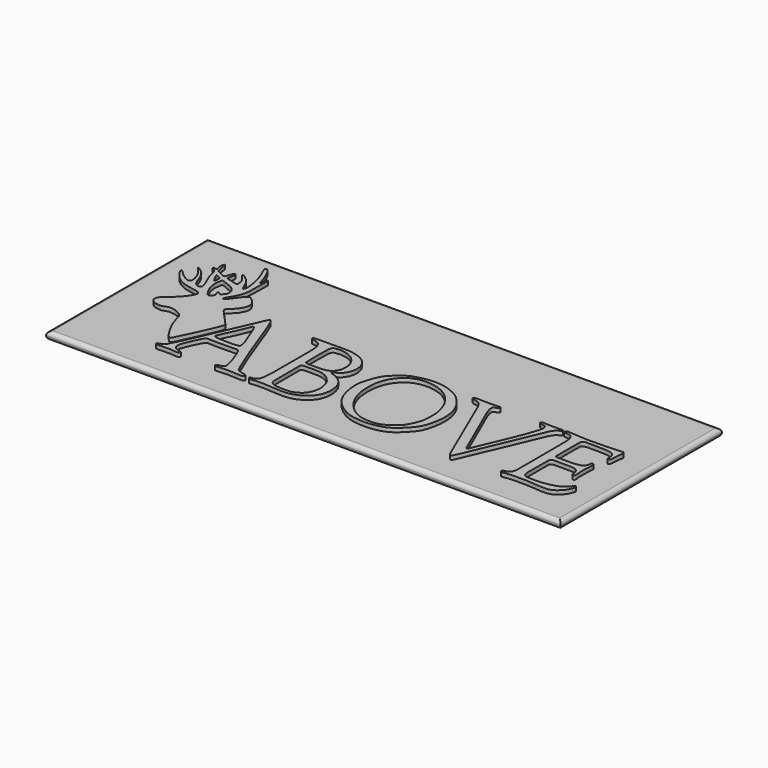
from build123d import *

# Parameters (mm, degrees)
F1_DEPTH = 0.4
F3_DEPTH = 2
F4_W     = 130.9761814773
F4_H     = 51.3558490202
F5_DEPTH = 1
F6_R     = 0.99999
F7_DEPTH = 2


# Not quite as in the source:
# - a fillet or chamfer is up to 0.001 mm smaller than in the source, because OpenCascade refuses the exact size


with BuildPart() as f1:
    # F0 (on Top) → F1 (new body)
    with BuildSketch(Plane.XY):
        with BuildLine():
            add(Edge.make_bspline(
                [(-15.2332797082, -10.2984596184), (-15.0093942884, -9.6524336301), (-15.0840574343, -9.1280532888), (-19.4655234335, -4.9444968794), (-19.1923468425, -4.0814513582), (-17.0227818195, -2.3777963682), (-15.9772713992, 0.6445409531), (-17.9010980306, 2.3727251331), (-19.2227726204, 3.4732306517), (-22.0102515264, -1.694371511), (-22.675957849, -0.7190837107), (-21.4698886603, 0.7632452243), (-20.1707249074, 3.6211502447), (-20.3340098043, 7.3677276696), (-20.0693177036, 11.1555273847), (-20.7490299306, 10.0046641789), (-20.7993278871, 7.9484959257), (-21.6196261476, 11.7801006923), (-23.3189903301, 14.5604952951), (-24.2268096177, 14.163796693), (-22.3143449492, 11.0669257332), (-21.331542924, 5.6400698523), (-22.149053501, 4.2936073138), (-22.8841040318, 7.5286045669), (-25.190165698, 9.3200917664), (-26.0899436297, 9.4842529604), (-24.1985357481, 7.5014652247), (-24.0857988599, 6.3361531301), (-24.1034586627, 5.3123553051), (-26.1386607352, 6.1357702948), (-27.122761487, 6.2654212324), (-27.2973682829, 6.6475846064), (-26.710529351, 8.7559265568), (-27.5771616457, 8.8747247494), (-27.9381930899, 6.9693446297), (-28.3530093382, 6.4188046355), (-30.1959305266, 7.4880147192), (-30.6145836041, 7.6246936128), (-31.1504494343, 9.4485056194), (-31.0918334587, 11.0700867085), (-31.8428582792, 9.7455582197), (-31.0093663734, 7.608908434), (-31.9606356015, 8.4144559492), (-32.5662439462, 7.9809408066), (-30.8829651102, 7.3675040083), (-31.1062693781, 5.1768624873), (-27.8910672871, -0.2497095271), (-31.266558052, 0.2817087175), (-31.6391364369, 4.8260598868), (-35.8656403415, 7.148054973), (-32.5956541042, 4.5606439482), (-31.5129435253, -0.6532739833), (-35.3555837278, 2.3321158484), (-35.5396776514, 2.6488410814), (-37.423089105, 4.3576754946), (-34.149133245, -1.644392368), (-27.3820098453, -1.2956673683), (-27.8794549907, -3.5887880219), (-30.3693556852, -6.6236284339), (-33.142877036, -8.3616003025), (-33.1843468192, -10.5862835101), (-29.9525050745, -11.479426381), (-28.7488139728, -10.1627989737), (-24.3130688974, -11.3403488056), (-24.3577602886, -14.9079605545), (-20.408517341, -21.5471299333), (-19.3708138898, -19.6570120394), (-15.8667838924, -12.1264489854), (-15.2332797082, -10.2984596184)],
                knots=[0, 0, 0, 0, 0.0120407609, 0.0369548453, 0.0455998656, 0.0626817696, 0.0806453343, 0.096699598, 0.1079623462, 0.131302389, 0.1377707175, 0.1515788078, 0.1702063006, 0.1919656057, 0.2094349262, 0.2180452799, 0.2292360252, 0.2468462896, 0.2660436632, 0.2722493285, 0.291374186, 0.316870226, 0.3253231285, 0.3424600791, 0.3610099087, 0.3669824396, 0.382641769, 0.394942166, 0.4030509241, 0.417573897, 0.4280639686, 0.4342264289, 0.4491088709, 0.4554393353, 0.4696299423, 0.4773554298, 0.4919040126, 0.4992434437, 0.5138107783, 0.5247485618, 0.5349387212, 0.5487104407, 0.5571075282, 0.5634453361, 0.5747861505, 0.5909866388, 0.6145658117, 0.6271821922, 0.6498661243, 0.6673736433, 0.6844679828, 0.7042723063, 0.7225110601, 0.7315999829, 0.7424569843, 0.7648776789, 0.7908505506, 0.8029463447, 0.824154807, 0.8430628881, 0.856291921, 0.8737242258, 0.8873169312, 0.907208903, 0.9275153958, 0.9544482361, 0.9659295704, 1, 1, 1, 1], degree=3))
        make_face()
        with BuildLine():
            add(Edge.make_bspline(
                [(-29.7977950352, 6.2162249849), (-29.7993964975, 6.0210812953), (-28.825569652, 3.8423834775), (-28.4519385095, 4.1422737352), (-28.3900703312, 5.1631622895), (-28.373725171, 5.5205005946), (-29.5818671337, 6.0474269447), (-29.7973504539, 6.2703987425), (-29.7977950352, 6.2162249849)],
                knots=[0, 0, 0, 0, 0.299300632, 0.3869764424, 0.5805649542, 0.6945409912, 0.9169112775, 1, 1, 1, 1], degree=3))
        make_face(mode=Mode.SUBTRACT)
        with BuildLine():
            add(Edge.make_bspline(
                [(-27.4534161738, 4.8815971646), (-27.5829006668, 4.6197704851), (-27.8833951504, 2.8656868488), (-27.3925534695, 0.799538413), (-26.4658323416, -0.8375371732), (-25.8457754123, -1.7123795224), (-25.2731466356, -1.7150173269), (-24.6325995931, -0.8642885968), (-24.6173490595, -0.6062435916), (-24.9744846122, 0.1084179836), (-24.9952901889, 0.8322824569), (-24.1482202231, 0.0273024167), (-23.7244798154, 0.3033967102), (-22.9372055408, 1.1829986707), (-23.0915123982, 2.4562011894), (-23.8408625303, 3.8662768208), (-26.9223285545, 4.8960420358), (-27.3223330185, 5.0270299743), (-27.4145706618, 4.9601455004), (-27.4534161738, 4.8815971646)],
                knots=[0, 0, 0, 0, 0.0817632462, 0.1726013597, 0.2550012881, 0.3138554901, 0.3543569034, 0.4137592441, 0.444060647, 0.4986368209, 0.5368103458, 0.5910850521, 0.630502456, 0.6931495414, 0.7578834718, 0.8336767969, 0.9399672197, 0.9754709225, 1, 1, 1, 1], degree=3))
        make_face(mode=Mode.SUBTRACT)
    extrude(amount=F1_DEPTH)


with BuildPart() as f3:
    # F2 (on Top) → F3 (new body)
    with BuildSketch(Plane.XY):
        with BuildLine():
            add(Edge.make_bspline(
                [(-17.8186707199, -24.5789550245), (-18.5262242711, -24.6304439452), (-20.358175603, -24.7394529453), (-20.7940909596, -24.4840161854), (-20.6337741479, -23.9779671505), (-19.3896907217, -23.8896324628), (-18.1771791891, -22.2724269857), (-9.970002365, -3.1502325051), (-9.4341293462, -2.1626326794), (-8.5298213567, -3.0073907103), (-6.1164796385, -10.2539467622), (-1.3806819347, -22.3025182489), (-0.683738408, -23.2547899839), (0.586258441, -23.6686196362), (1.6564266278, -23.8527715304), (1.9065968781, -24.3190250875), (1.4282647943, -24.8392161885), (-2.5654340217, -24.2992923004), (-5.0926669543, -24.6635461429), (-5.6461058536, -24.609920481), (-5.8601113726, -24.1039841591), (-4.9881206956, -23.8322315995), (-4.0057600347, -23.7565204031), (-3.7041440652, -22.3979584639), (-5.970768949, -16.3593958047), (-6.6672962176, -16.3671332574), (-13.9351018709, -16.5336977205), (-14.4412111372, -16.1030933493), (-17.1251492443, -21.5812553775), (-16.8820571682, -23.0099438036), (-16.3728003844, -23.6025789105), (-15.1423881637, -24.1280540106), (-14.5677091572, -24.0823658212), (-14.4953555678, -24.9679629884), (-16.8880971826, -24.4933044304), (-17.3513145138, -24.544945349), (-17.8186707199, -24.5789550245)],
                knots=[0, 0, 0, 0, 0.034606547, 0.0478551254, 0.0607316403, 0.0815592174, 0.1138190862, 0.2124412902, 0.2309948002, 0.2485416257, 0.3094963798, 0.3875252451, 0.409110504, 0.433162012, 0.4555813572, 0.4688299488, 0.4829975336, 0.5262737256, 0.5615253264, 0.5756929131, 0.588282433, 0.6072660436, 0.6274333282, 0.6509110315, 0.7042405462, 0.7242470082, 0.7812023235, 0.7974767625, 0.8486624145, 0.8746413843, 0.8926317285, 0.9174233866, 0.9324998026, 0.9465406554, 0.9771415401, 1, 1, 1, 1], degree=3))
        make_face()
        with BuildLine():
            add(Edge.make_bspline(
                [(-10.6451269239, -7.6531427912), (-11.1635320486, -9.140155094), (-13.5771506003, -13.9866832023), (-13.6553005281, -14.612677821), (-13.1015114277, -15.08954204), (-6.8594531157, -15.1835333702), (-7.1281559565, -14.448692861), (-7.09391842, -13.2187966821), (-8.656445023, -9.9815808182), (-9.7266075902, -6.5997926543), (-10.4475039943, -6.7365001924), (-10.4546387692, -7.1067395708), (-10.6451269239, -7.6531427912)],
                knots=[0, 0, 0, 0, 0.1955711938, 0.2489704346, 0.3074664099, 0.4860203681, 0.5291103449, 0.6060239634, 0.7520174877, 0.8858844196, 0.9281372925, 1, 1, 1, 1], degree=3))
        make_face(mode=Mode.SUBTRACT)
    extrude(amount=F3_DEPTH)


with BuildPart() as f3b:
    # F2 (on Top) → F3, piece 2 (new body)
    with BuildSketch(Plane.XY):
        with BuildLine():
            add(Edge.make_bspline(
                [(2.9986717273, -2.9176652897), (4.5731932325, -2.8947406218), (10.9523054272, -2.8056420795), (11.8491369393, -2.9704794263), (15.1441637743, -3.7111802915), (17.1291392253, -5.973921605), (17.4434691373, -8.7077246139), (16.351884791, -11.3349808797), (14.4830876864, -12.0868741598), (14.2065407888, -12.6919101169), (15.3907005999, -12.7503578443), (18.0051408366, -14.3724783841), (18.9323318972, -16.612656188), (19.2045201156, -19.8438815811), (17.5618176451, -22.9328146445), (14.4991929645, -24.5620027924), (11.9328529247, -24.9275981507), (8.0759131802, -24.6237266642), (5.2376508672, -24.4574170198), (3.4847200578, -24.7552756049), (3.000104703, -24.6856083566), (2.840094494, -24.2661535545), (3.1077172317, -23.9845093652), (3.7233931441, -24.1261225507), (4.8130212078, -23.4964830947), (5.1143694454, -21.7499883345), (5.2795577601, -18.7920313061), (5.093980589, -12.2053829442), (5.3207697442, -7.2503768517), (4.9675852293, -5.2741108501), (4.518908773, -4.3142462301), (3.4077663416, -3.6151473735), (2.4609358883, -3.7162434327), (2.047195786, -3.4704848142), (2.1544159455, -2.9304379219), (2.4815498265, -2.9251944646), (2.9986717273, -2.9176652897)],
                knots=[0, 0, 0, 0, 0.0594003701, 0.0835026048, 0.1206841975, 0.1572307632, 0.1917765774, 0.2270665321, 0.256394898, 0.2691563441, 0.2892990909, 0.3263944414, 0.3595571245, 0.3971334828, 0.4362595917, 0.4749411121, 0.5094013726, 0.5512949807, 0.5882689746, 0.6158124967, 0.6294268394, 0.6421580801, 0.6537191257, 0.6698855437, 0.6922755626, 0.7193150847, 0.7560647655, 0.811759297, 0.8599220026, 0.8888715544, 0.9100993257, 0.9338553359, 0.9544697139, 0.9676822069, 0.9804910684, 1, 1, 1, 1], degree=3))
        make_face()
        with BuildLine():
            add(Edge.make_bspline(
                [(7.9134525731, -13.5765336454), (8.4656908215, -13.5249837722), (12.0166451852, -13.482074654), (13.1072424292, -13.7143378792), (14.509090113, -14.3336197357), (15.6591165801, -15.5440421064), (16.1790934207, -16.2740694615), (16.7715367956, -18.0506637137), (16.81110186, -19.5984971483), (16.3535796726, -21.4566097884), (15.4796202328, -22.7291384826), (13.9450284962, -23.653515414), (12.4734478276, -24.0015308029), (9.9325274889, -23.9052985449), (8.9655494456, -23.7359270018), (8.2751637862, -23.4966310779), (7.5920920663, -22.8790822924), (7.5227255198, -21.8494720153), (7.5755301319, -17.2633260081), (7.5553347596, -14.0348315189), (7.5658004299, -13.885882511), (7.708510426, -13.617057364), (7.7812264073, -13.5888765827), (7.9134525731, -13.5765336454)],
                knots=[0, 0, 0, 0, 0.0796721885, 0.1263040133, 0.1742904671, 0.225547667, 0.2640510909, 0.3176224, 0.3685996925, 0.4231997985, 0.472914118, 0.5250153616, 0.5755784316, 0.6391972187, 0.6790868472, 0.7126185496, 0.7487122899, 0.7874658877, 0.8765007975, 0.9467593746, 0.960892758, 0.9809235452, 1, 1, 1, 1], degree=3))
        make_face(mode=Mode.SUBTRACT)
        with BuildLine():
            add(Edge.make_bspline(
                [(7.5597460382, -5.1983157173), (7.5768174771, -4.7752658686), (7.6117939175, -4.5599184391), (7.8915823244, -3.9518990986), (8.5512243646, -3.7987113384), (9.6421145995, -3.6374130657), (12.0142479626, -4.0121152092), (13.9056770375, -5.3663836659), (15.0189228434, -7.2511220165), (15.1903015952, -9.0285684555), (14.9912671632, -10.3350820672), (14.3210946635, -11.493000004), (13.0422817282, -12.5872460163), (8.3767248185, -12.4282745943), (7.9626085673, -12.42584987), (7.6082300578, -12.2055804985), (7.4622628161, -11.7055791022), (7.5083058526, -6.4730625476), (7.5597460382, -5.1983157173)],
                knots=[0, 0, 0, 0, 0.04366644, 0.0812507687, 0.1215889048, 0.1754155404, 0.2545074138, 0.3331504508, 0.4083572449, 0.4764587283, 0.5350867206, 0.5920341657, 0.6594086428, 0.7688242446, 0.8023163354, 0.8306341757, 0.8684229384, 1, 1, 1, 1], degree=3))
        make_face(mode=Mode.SUBTRACT)
    extrude(amount=F3_DEPTH)


with BuildPart() as f3c:
    # F2 (on Top) → F3, piece 3 (new body)
    with BuildSketch(Plane.XY):
        with BuildLine():
            add(Edge.make_bspline(
                [(31.6981896758, -2.7517566923), (32.4855511917, -2.6662951361), (33.6973140893, -2.686447277), (35.4124903207, -2.8976716178), (37.365271922, -3.487745744), (39.7322577308, -4.6286347181), (41.7448723321, -6.7403695787), (42.9307226187, -8.5981241795), (43.7743743926, -11.0623168107), (44.0310311172, -14.1276205282), (43.2370107981, -18.0437680394), (42.1417511843, -20.2200499423), (39.0584845813, -23.3581879437), (36.6879540703, -24.4147562849), (33.547977925, -25.0431152226), (29.8149106979, -24.7845936888), (27.2978257333, -24.0149400802), (24.1855473843, -21.8152677053), (22.3600004098, -19.1779329614), (21.4690708366, -15.8722935856), (21.327289014, -13.3523817345), (21.5138448111, -11.6902719815), (22.6387088646, -8.2258594008), (23.7475713067, -6.6545022043), (26.1812598582, -4.3383661288), (28.3603805442, -3.356356178), (30.6942257638, -2.8607286405), (31.6981896758, -2.7517566923)],
                knots=[0, 0, 0, 0, 0.0341965483, 0.0650580209, 0.0990248333, 0.1379292236, 0.1785675923, 0.2140382543, 0.2519077228, 0.2943765314, 0.34143948, 0.3795504523, 0.428692638, 0.4674522524, 0.5099281851, 0.5559166818, 0.5949378648, 0.6407882758, 0.6838578711, 0.7280535962, 0.765304292, 0.7967660624, 0.8414591274, 0.8758812293, 0.9184921551, 0.9563960141, 1, 1, 1, 1], degree=3))
        make_face()
        with BuildLine():
            add(Edge.make_bspline(
                [(32.3757380247, -3.7556143943), (33.2958323259, -3.835045558), (35.3374829386, -4.2298619022), (37.8702307643, -5.7717201967), (39.5353026217, -7.7515539991), (40.6118543591, -9.4957685202), (41.3311781149, -11.9217308369), (41.537384592, -13.2175494886), (41.5631804343, -16.024805783), (41.3191550954, -17.6196524909), (40.0632173963, -20.4459911485), (39.0176525098, -21.7261039941), (36.4226916998, -23.6310371312), (34.2590014297, -24.0790860379), (31.240481395, -23.9596385587), (29.4134002337, -23.1742800285), (27.5909988603, -22.0154832916), (25.8072628968, -19.8685430648), (24.9790822222, -18.3822532534), (24.1095178811, -16.0311551863), (23.9312299748, -14.4145168967), (23.7957549823, -12.4832029945), (23.9334985957, -10.5232236657), (24.6149450631, -8.233839022), (25.2694976229, -7.0783307387), (26.3486933371, -5.6845001426), (27.7015348542, -4.5304110567), (30.0674452085, -3.7306413055), (31.5570074754, -3.6849338998), (32.3757380247, -3.7556143943)],
                knots=[0, 0, 0, 0, 0.0429022088, 0.0858322177, 0.1254390468, 0.1616438754, 0.200344307, 0.2299741373, 0.2705942497, 0.3038292435, 0.3463741966, 0.3795926892, 0.4230236918, 0.4608566752, 0.5034618232, 0.5384774913, 0.5750783278, 0.6162288942, 0.6495270762, 0.6883054272, 0.720542142, 0.7546314557, 0.7902429882, 0.8283403313, 0.8573019616, 0.8897134595, 0.9230753544, 0.9618241859, 1, 1, 1, 1], degree=3))
        make_face(mode=Mode.SUBTRACT)
    extrude(amount=F3_DEPTH)


with BuildPart() as f3d:
    # F2 (on Top) → F3, piece 4 (new body)
    with BuildSketch(Plane.XY):
        with BuildLine():
            add(Edge.make_bspline(
                [(43.4478521587, -3.0493328889), (44.5846660798, -3.1063553315), (46.6244936083, -3.2085442718), (49.4442464963, -3.0121823146), (49.8430234234, -3.0347621192), (50.0485700829, -3.3512100722), (49.7660583429, -3.674682885), (49.3274870978, -3.7871947915), (48.8139123394, -4.0140117338), (48.5980931136, -4.4175614975), (48.7332427344, -5.3460822505), (49.3050834915, -6.9306989902), (51.1307713098, -10.9088610465), (55.2860542634, -20.5594377099), (55.3790988692, -20.7607972863), (55.3798365892, -20.760195779), (55.4215515437, -20.8339544375)],
                knots=[0, 0, 0, 0, 0.1188220262, 0.2237195129, 0.2608396256, 0.2948710905, 0.3332159131, 0.3773807578, 0.424501898, 0.4653824938, 0.5249451089, 0.6028688594, 0.749352672, 0.9539072272, 0.97311764, 0.9946758844, 0.9946758844, 0.9946758844, 0.9946758844], degree=3))
            add(Edge.make_bspline(
                [(55.4607037074, -20.9034150784), (55.4866189211, -20.9430088187), (55.5388381616, -21.022790335), (55.6560705125, -21.1784298749), (55.9305236933, -20.9984367057), (56.1392833118, -20.5234944666), (56.3837353272, -20.0621710379), (58.4718341466, -14.9666961091), (60.3944590747, -10.6123481531), (61.7502440603, -6.8328535787), (62.0979632028, -5.5929443597), (62.1938028184, -4.7472395828), (62.1227279981, -4.2320286696), (61.8320675007, -3.8800678569), (61.3656773155, -3.7644159671), (60.5629669431, -3.6089124364), (60.3459094201, -3.4920842872), (60.1055323717, -3.3316895125), (60.1372555353, -3.1150390963), (60.3239178294, -2.9576815651), (60.7711186994, -2.9102152421), (62.4420232453, -3.1033594688), (65.5839100323, -3.002560101), (65.6363353042, -2.9806084462), (65.9109486239, -3.081184096), (65.8590357012, -3.5015165095), (65.3542516668, -3.587012591), (64.4140603578, -4.2094095114), (63.7112014267, -5.5838872142), (62.804680902, -7.8958159046), (60.2703107713, -13.7714791057), (58.891988443, -17.0987199578), (57.4604076229, -20.3876905791), (55.9606004977, -23.932193809), (55.6045347914, -24.8074523644), (55.3690455445, -25.2644164156), (55.0818956105, -25.4798132289), (54.7062400575, -25.3298895913), (54.358648808, -24.742624418), (53.1783713435, -21.884382719), (52.1770231081, -19.5366299305), (51.0835176671, -17.0092270696), (49.7964172999, -14.04326035), (48.3314159163, -10.6108341908), (46.9299138991, -7.3547336689), (45.9859771758, -5.1659938333), (45.4431505429, -4.4583801964), (44.8930013483, -4.0178146836), (44.3657666742, -3.8838703949), (43.721768661, -3.7882978412), (43.2686629705, -3.6332026634), (43.1462142801, -3.5755733492), (43.0385249855, -3.2680682596), (43.2752626563, -3.0655793599), (43.3950395425, -3.0543043306), (43.4478521587, -3.0493328889)],
                knots=[0, 0, 0, 0, 0.0069195808, 0.0139429779, 0.0232181225, 0.0357670809, 0.048423783, 0.0893876317, 0.1316102802, 0.1668085072, 0.1869548417, 0.2030729985, 0.2158274826, 0.2272557348, 0.2399557033, 0.2561310963, 0.2653567827, 0.2743797104, 0.2820397862, 0.2903830247, 0.3012570035, 0.3261470545, 0.3574257754, 0.3617631056, 0.3703785591, 0.3804125429, 0.3925272533, 0.4112135027, 0.4329087196, 0.461589806, 0.5071989225, 0.5420687864, 0.5766617428, 0.6117707112, 0.6288917885, 0.6412497336, 0.6513234957, 0.6615107064, 0.6757756137, 0.7071612792, 0.7369589923, 0.7664511377, 0.7988955327, 0.8340077468, 0.8685372617, 0.8958968437, 0.9125277557, 0.9271130859, 0.9403499786, 0.9551753729, 0.9673602344, 0.9737678566, 0.983189181, 0.9925876907, 1, 1, 1, 1], degree=3))
            add(Edge.make_bspline(
                [(55.4215515437, -20.8339544375), (55.4318536462, -20.8521701892), (55.4446762067, -20.8749039801), (55.4607037074, -20.9034150784)],
                knots=[0.9946758844, 0.9946758844, 0.9946758844, 0.9946758844, 1, 1, 1, 1], degree=3))
        make_face()
    extrude(amount=F3_DEPTH)


with BuildPart() as f3e:
    # F2 (on Top) → F3, piece 5 (new body)
    with BuildSketch(Plane.XY):
        with BuildLine():
            add(Edge.make_bspline(
                [(67.0425593853, -2.8810673393), (67.8678731279, -2.938649076), (72.7499173271, -3.4609926409), (80.755809882, -2.9446053024), (80.9969352571, -2.8768406134), (81.5035604288, -3.2620983162), (81.1373324461, -4.1403665714), (81.1141305135, -5.9013244473), (81.0144246811, -6.8806777807), (80.8788745766, -7.256085935), (80.5697803911, -7.3310123724), (80.2202021226, -7.1464714359), (80.3569655259, -6.4328912197), (80.213063495, -5.5770025247), (79.8116923244, -4.9059892697), (79.059082448, -4.4485175303), (77.5400597323, -4.2958692153), (75.9115890583, -4.2759782621), (72.8491726424, -4.2357289919), (72.2369273298, -4.3102226833), (71.7266219665, -4.5612120941), (71.5870798919, -5.2364526317), (71.6168007769, -6.4715093591), (71.5883648454, -12.2308260651), (71.6448754233, -12.5722157719), (71.8098561835, -12.8893748688), (72.3879462029, -12.8936691788), (75.2234716277, -12.9140276015), (76.840911265, -12.8735885729), (78.0156862933, -12.614818358), (78.6282283257, -12.4164568074), (78.9786760033, -11.5075158323), (79.0521986523, -10.9581593735), (79.1460235667, -10.6244449846), (79.5289645607, -10.5165075494), (79.8442025902, -10.8101021592), (79.7044768444, -11.8424237925), (79.6403669336, -12.8637636298), (79.5814672022, -14.7758326897), (79.7581782043, -16.3464053921), (79.7613391422, -16.7260706296), (79.5123768635, -16.9163637614), (79.1014232124, -16.8026333448), (79.0368955978, -16.3168696512), (78.8675268978, -15.5233552201), (78.5828850376, -14.8361243406), (77.7468299272, -14.4096002438), (77.2761877315, -14.260780277), (72.5789593252, -14.2071704853), (72.1044236508, -14.3344197004), (71.6693041261, -14.4657576895), (71.5887169569, -15.0676546067), (71.6647372618, -15.5918118463), (71.4734106503, -21.7739564846), (71.7553651667, -22.4942609751), (71.9281879782, -22.934195017), (72.4703722946, -23.2052113809), (73.903085566, -23.3616238483), (76.167290383, -23.3124131308), (78.4205079795, -22.9981859312), (80.0384450974, -22.4719900357), (81.0238499912, -21.9238236424), (81.9290842616, -21.2272537598), (82.3910465155, -20.4543088275), (82.6606264627, -20.1894802427), (83.0216396451, -20.3408452951), (83.0245155059, -20.9665332697), (82.6622045973, -22.0354600319), (81.7777847881, -23.3181111603), (80.4043746409, -24.4380276617), (79.0902431356, -24.8262221852), (77.1906087385, -24.7494223836), (75.4969237861, -24.5669595686), (73.0438507514, -24.419721641), (71.2751820322, -24.4452149202), (69.2893380169, -24.4781183856), (68.007343532, -24.7174323227), (67.4504717694, -24.7572667737), (67.0946462472, -24.6285520287), (67.0513295884, -24.2109980974), (67.4496485866, -23.9715317476), (68.4378505535, -23.8480031872), (69.0421296121, -23.1353918146), (69.2481758301, -22.125989542), (69.224139086, -21.0294021349), (69.2369444617, -15.9647527894), (69.2322017281, -11.3690933247), (69.2345551924, -6.7204678383), (69.1824960235, -5.8656391962), (68.9000729874, -4.4857074747), (68.3837412389, -3.9329285101), (67.5968850774, -3.6199891404), (66.887460842, -3.6097702489), (66.4840789118, -3.5986137844), (66.2793742262, -3.3283120521), (66.5768836391, -2.8617867493), (66.8094482842, -2.8648032917), (67.0425593853, -2.8810673393)],
                knots=[0, 0, 0, 0, 0.0246056079, 0.0530652917, 0.0575288415, 0.0643933714, 0.0738209208, 0.0875455486, 0.0976388121, 0.1035084775, 0.1087720979, 0.1143580091, 0.12257523, 0.1321248493, 0.140850639, 0.1500886786, 0.1622124883, 0.1759187448, 0.1934463296, 0.201431505, 0.2084304197, 0.2159388738, 0.2281401034, 0.2522733021, 0.2583326284, 0.2634475908, 0.27063428, 0.2876863466, 0.3012387286, 0.3119498758, 0.3197697021, 0.329448883, 0.337145219, 0.3427460764, 0.3485052844, 0.3543591621, 0.3642924285, 0.3748301525, 0.3890910899, 0.4017961391, 0.4075465, 0.4126614547, 0.4186038511, 0.4253641982, 0.4345504776, 0.4433063026, 0.4524075821, 0.4604495602, 0.4821275863, 0.4897842144, 0.4958172395, 0.5028411307, 0.5110573447, 0.5360536144, 0.5453571943, 0.5515484458, 0.558963169, 0.570960721, 0.5864452307, 0.6018975569, 0.6149657881, 0.625653872, 0.6364862087, 0.646054903, 0.6517745124, 0.6571270049, 0.6645771952, 0.6753164104, 0.6880748021, 0.7013909137, 0.7131600094, 0.7268637203, 0.7403692179, 0.7560862548, 0.769821435, 0.7841188305, 0.7956422494, 0.8030278605, 0.8087633767, 0.8145137307, 0.8209594683, 0.8309286631, 0.8404799772, 0.8503060805, 0.8607910857, 0.8830397741, 0.9063335685, 0.9273831296, 0.9369743944, 0.9485193988, 0.957244373, 0.9664032559, 0.9749943578, 0.9812037123, 0.9863437118, 0.9930501093, 1, 1, 1, 1], degree=3))
        make_face()
    extrude(amount=F3_DEPTH)


with BuildPart() as f5:
    # F4 (on Top) → F5 (new body, symmetric)
    with BuildSketch(Plane.XY):
        with Locations((23.1191609055, -6.7132958211)):
            Rectangle(F4_W, F4_H)
    extrude(amount=F5_DEPTH, both=True)

    # F6 (radius 1 in the source; OpenCascade refuses exactly that, so slightly less here)
    f6_edges = [f5.edges().sort_by_distance(p)[0] for p in [
        (23.119161, -32.39122, 1),
        (88.607252, -6.713296, 1),
        (23.119161, 18.964629, 1),
        (-42.36893, -6.713296, 1),
        (23.119161, -32.39122, -1),
        (88.607252, -6.713296, -1),
        (23.119161, 18.964629, -1),
        (-42.36893, -6.713296, -1),
    ]]
    fillet(f6_edges, radius=F6_R)


with BuildPart() as f7:
    # F0 (on Top) → F7 (new body)
    with BuildSketch(Plane.XY):
        with BuildLine():
            add(Edge.make_bspline(
                [(-15.2332797082, -10.2984596184), (-15.0093942884, -9.6524336301), (-15.0840574343, -9.1280532888), (-19.4655234335, -4.9444968794), (-19.1923468425, -4.0814513582), (-17.0227818195, -2.3777963682), (-15.9772713992, 0.6445409531), (-17.9010980306, 2.3727251331), (-19.2227726204, 3.4732306517), (-22.0102515264, -1.694371511), (-22.675957849, -0.7190837107), (-21.4698886603, 0.7632452243), (-20.1707249074, 3.6211502447), (-20.3340098043, 7.3677276696), (-20.0693177036, 11.1555273847), (-20.7490299306, 10.0046641789), (-20.7993278871, 7.9484959257), (-21.6196261476, 11.7801006923), (-23.3189903301, 14.5604952951), (-24.2268096177, 14.163796693), (-22.3143449492, 11.0669257332), (-21.331542924, 5.6400698523), (-22.149053501, 4.2936073138), (-22.8841040318, 7.5286045669), (-25.190165698, 9.3200917664), (-26.0899436297, 9.4842529604), (-24.1985357481, 7.5014652247), (-24.0857988599, 6.3361531301), (-24.1034586627, 5.3123553051), (-26.1386607352, 6.1357702948), (-27.122761487, 6.2654212324), (-27.2973682829, 6.6475846064), (-26.710529351, 8.7559265568), (-27.5771616457, 8.8747247494), (-27.9381930899, 6.9693446297), (-28.3530093382, 6.4188046355), (-30.1959305266, 7.4880147192), (-30.6145836041, 7.6246936128), (-31.1504494343, 9.4485056194), (-31.0918334587, 11.0700867085), (-31.8428582792, 9.7455582197), (-31.0093663734, 7.608908434), (-31.9606356015, 8.4144559492), (-32.5662439462, 7.9809408066), (-30.8829651102, 7.3675040083), (-31.1062693781, 5.1768624873), (-27.8910672871, -0.2497095271), (-31.266558052, 0.2817087175), (-31.6391364369, 4.8260598868), (-35.8656403415, 7.148054973), (-32.5956541042, 4.5606439482), (-31.5129435253, -0.6532739833), (-35.3555837278, 2.3321158484), (-35.5396776514, 2.6488410814), (-37.423089105, 4.3576754946), (-34.149133245, -1.644392368), (-27.3820098453, -1.2956673683), (-27.8794549907, -3.5887880219), (-30.3693556852, -6.6236284339), (-33.142877036, -8.3616003025), (-33.1843468192, -10.5862835101), (-29.9525050745, -11.479426381), (-28.7488139728, -10.1627989737), (-24.3130688974, -11.3403488056), (-24.3577602886, -14.9079605545), (-20.408517341, -21.5471299333), (-19.3708138898, -19.6570120394), (-15.8667838924, -12.1264489854), (-15.2332797082, -10.2984596184)],
                knots=[0, 0, 0, 0, 0.0120407609, 0.0369548453, 0.0455998656, 0.0626817696, 0.0806453343, 0.096699598, 0.1079623462, 0.131302389, 0.1377707175, 0.1515788078, 0.1702063006, 0.1919656057, 0.2094349262, 0.2180452799, 0.2292360252, 0.2468462896, 0.2660436632, 0.2722493285, 0.291374186, 0.316870226, 0.3253231285, 0.3424600791, 0.3610099087, 0.3669824396, 0.382641769, 0.394942166, 0.4030509241, 0.417573897, 0.4280639686, 0.4342264289, 0.4491088709, 0.4554393353, 0.4696299423, 0.4773554298, 0.4919040126, 0.4992434437, 0.5138107783, 0.5247485618, 0.5349387212, 0.5487104407, 0.5571075282, 0.5634453361, 0.5747861505, 0.5909866388, 0.6145658117, 0.6271821922, 0.6498661243, 0.6673736433, 0.6844679828, 0.7042723063, 0.7225110601, 0.7315999829, 0.7424569843, 0.7648776789, 0.7908505506, 0.8029463447, 0.824154807, 0.8430628881, 0.856291921, 0.8737242258, 0.8873169312, 0.907208903, 0.9275153958, 0.9544482361, 0.9659295704, 1, 1, 1, 1], degree=3))
        make_face()
        with BuildLine():
            add(Edge.make_bspline(
                [(-29.7977950352, 6.2162249849), (-29.7993964975, 6.0210812953), (-28.825569652, 3.8423834775), (-28.4519385095, 4.1422737352), (-28.3900703312, 5.1631622895), (-28.373725171, 5.5205005946), (-29.5818671337, 6.0474269447), (-29.7973504539, 6.2703987425), (-29.7977950352, 6.2162249849)],
                knots=[0, 0, 0, 0, 0.299300632, 0.3869764424, 0.5805649542, 0.6945409912, 0.9169112775, 1, 1, 1, 1], degree=3))
        make_face(mode=Mode.SUBTRACT)
        with BuildLine():
            add(Edge.make_bspline(
                [(-27.4534161738, 4.8815971646), (-27.5829006668, 4.6197704851), (-27.8833951504, 2.8656868488), (-27.3925534695, 0.799538413), (-26.4658323416, -0.8375371732), (-25.8457754123, -1.7123795224), (-25.2731466356, -1.7150173269), (-24.6325995931, -0.8642885968), (-24.6173490595, -0.6062435916), (-24.9744846122, 0.1084179836), (-24.9952901889, 0.8322824569), (-24.1482202231, 0.0273024167), (-23.7244798154, 0.3033967102), (-22.9372055408, 1.1829986707), (-23.0915123982, 2.4562011894), (-23.8408625303, 3.8662768208), (-26.9223285545, 4.8960420358), (-27.3223330185, 5.0270299743), (-27.4145706618, 4.9601455004), (-27.4534161738, 4.8815971646)],
                knots=[0, 0, 0, 0, 0.0817632462, 0.1726013597, 0.2550012881, 0.3138554901, 0.3543569034, 0.4137592441, 0.444060647, 0.4986368209, 0.5368103458, 0.5910850521, 0.630502456, 0.6931495414, 0.7578834718, 0.8336767969, 0.9399672197, 0.9754709225, 1, 1, 1, 1], degree=3))
        make_face(mode=Mode.SUBTRACT)
    extrude(amount=F7_DEPTH)


solid = Compound([f1.part, f3.part, f3b.part, f3c.part, f3d.part, f3e.part, f5.part, f7.part])
